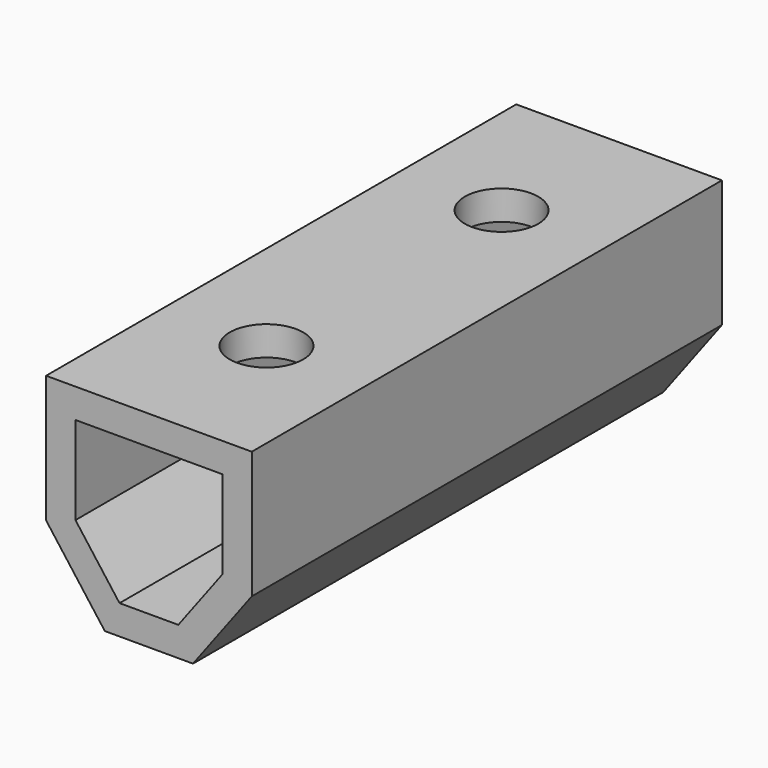
from build123d import *

# Parameters (mm, degrees)
F1_DEPTH = 10
F2_R     = 1.25
F3_DEPTH = 1


# Not quite as in the source:
# - ends of sketch curves that miss each other by under 0.0002 mm in the source are joined


with BuildPart() as f1:
    # F0 (on Front) → F1 (new body)
    with BuildSketch(Plane.XZ):
        Polygon((3.5, 6), (-3.4999988526, 6), (-3.5, 1.6666666667), (-1.5, -1), (0, -1), (1.5, -1), (3.5, 1.6666666667), align=None)
        Polygon((-2.5, 5), (0, 5), (2.5, 5), (2.5, 2), (1, 0), (0, 0), (-1, 0), (-2.5, 2), align=None, mode=Mode.SUBTRACT)
    extrude(amount=F1_DEPTH)

    # F2 (on face) → F3 (cut, through all)
    with BuildSketch(Plane.XY.offset(6)):
        with Locations((5.737e-07, -5)):
            Circle(F2_R)
    extrude(amount=-F3_DEPTH, mode=Mode.SUBTRACT)

    # F4: F1 across face


with BuildPart() as f1_1:
    add(f1.part)
    add(f1.part.mirror(Plane(origin=(4.016e-07, 0, 2.8888886977), x_dir=(1, 0, 0), z_dir=(0, 1, 0))))


solid = f1_1.part
